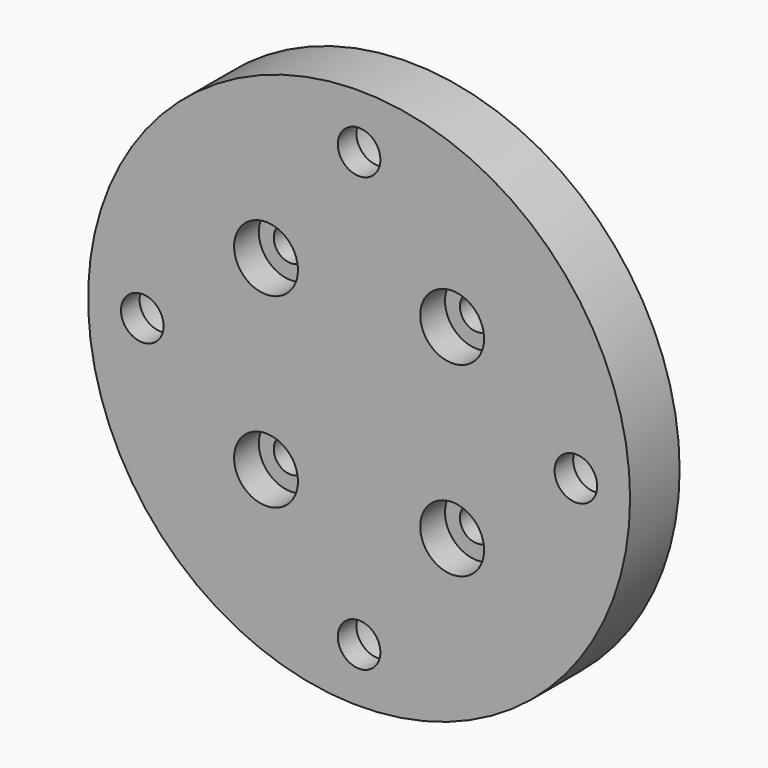
from build123d import *

# Parameters (mm, degrees)
F0_R            = 35
F0_R_2          = 14
F1_DEPTH        = 8
F2_DEPTH        = 4
F4_D            = 4.4
F4_CBORE_D      = 8.25
F4_CBORE_DEPTH  = 4
F4_COPIES_COUNT = 4
F5_D            = 5.5
F5_CBORE_D      = 9.75
F5_CBORE_DEPTH  = 5
F5_COPIES_COUNT = 4


# Not quite as in the source:
# - a pattern or mirror of a feature is missing from the dataset's text; its kind, count and spacing are read off the source's solid


with BuildPart() as f1:
    # F0 (on Front) → F1 (new body)
    with BuildSketch(Plane.XZ):
        Circle(F0_R)
        Circle(F0_R_2, mode=Mode.SUBTRACT)
        Circle(F0_R_2)
    extrude(amount=F1_DEPTH)

    # F0 (on Front) → F2 (join)
    with BuildSketch(Plane.XZ):
        Circle(F0_R_2)
    extrude(amount=-F2_DEPTH)

    # F4 (through all)
    with Locations(Plane.XZ.offset(8)):
        with Locations((12.0208152802, 12.0208152802)):
            f4 = CounterBoreHole(F4_D / 2, F4_CBORE_D / 2, F4_CBORE_DEPTH)

    # F4_copies: F4 ×4 about axis
    f4_copies_axis = Axis((0, 0, 0), (0, 1, 0))
    for i in range(1, F4_COPIES_COUNT):
        add(f4.rotate(f4_copies_axis, i * 360 / F4_COPIES_COUNT), mode=Mode.SUBTRACT)

    # F5 (through all)
    with Locations(Plane(origin=(0, 0, 0), x_dir=(1, 0, 0), z_dir=(0, 1, 0))):
        with Locations((0, -28)):
            f5 = CounterBoreHole(F5_D / 2, F5_CBORE_D / 2, F5_CBORE_DEPTH)

    # F5_copies: F5 ×4 about axis
    f5_copies_axis = Axis((0, 0, 0), (0, 1, 0))
    for i in range(1, F5_COPIES_COUNT):
        add(f5.rotate(f5_copies_axis, i * 360 / F5_COPIES_COUNT), mode=Mode.SUBTRACT)


solid = f1.part
